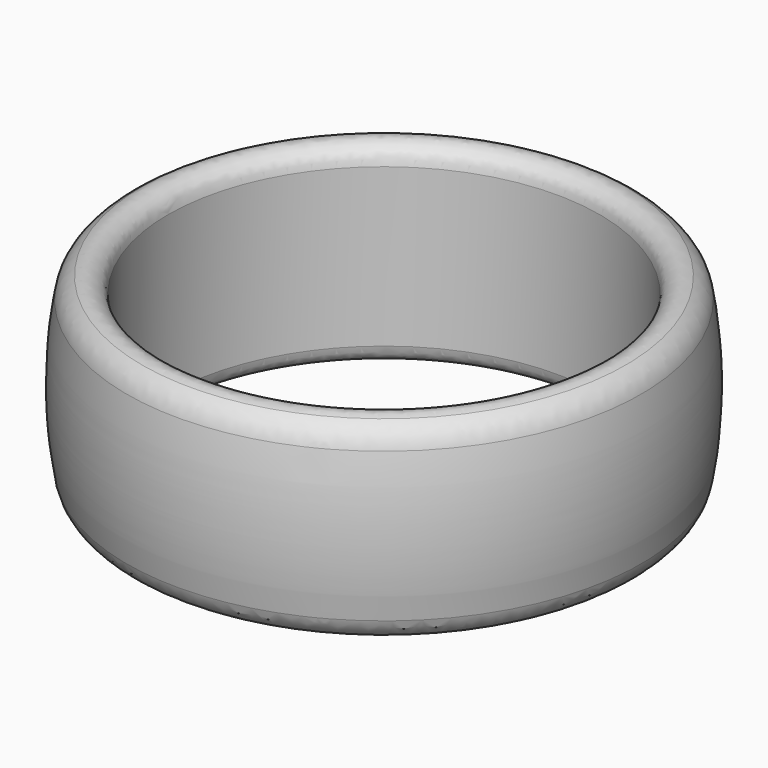
from build123d import *

# Parameters (mm, degrees)
F0_R          = 9
F1_DEPTH      = 5
F4_R          = 1.2
F5_R          = 0.75
F8_W          = 4.5
F8_H          = 1
F8_W_2        = 1
F8_H_2        = 4.5
F9_DEPTH      = 6.4
F10_TEXT_SIZE = 5.5555555556
F11_DEPTH     = 1
F12_TEXT_SIZE = 5.5555555556
F13_DEPTH     = 1
F14_TEXT_SIZE = 5.5555555556
F15_DEPTH     = 1


# Not quite as in the source:
# - Text() gives the source's letters only with a copy of the font that has no kerning and outlines rounded to 1/6400 em; it was checked with that copy


with BuildPart() as f1:
    # F0 (on Top) → F1 (new body)
    with BuildSketch(Plane.XY):
        Circle(F0_R)
    extrude(amount=F1_DEPTH)


with BuildPart() as f3:
    # F2 (on Front) → F3 (revolve)
    with BuildSketch(Plane.XZ):
        with BuildLine():
            Line((-10.5, 0), (-9, 0))
            Line((-9, 0), (-9, 8.1769345951))
            Line((-9, 8.1769345951), (-10.5, 8.1769345951))
            add(Edge.make_bspline(
                [(-10.5, 8.1769345951), (-11.6867599635, 4.0884672976), (-10.5, 0)],
                knots=[0.8438243034, 0.8438243034, 0.8438243034, 2.2977683502, 2.2977683502, 2.2977683502], degree=2, weights=[1, 0.7471902488, 1]))
        make_face()
    revolve(axis=Axis((0, 0, 0), (0, 0, -1)))

    # F4
    f4_edges = [f3.edges().sort_by_distance(p)[0] for p in [
        (10.5, 0, 8.176935),
        (10.5, 0, 0),
    ]]
    fillet(f4_edges, radius=F4_R)

    # F5
    f5_edges = [f3.edges().sort_by_distance(p)[0] for p in [
        (9, 0, 0),
        (9, 0, 8.176935),
    ]]
    fillet(f5_edges, radius=F5_R)

    # F8 (on offset) → F9 (join)
    with BuildSketch(Plane.XY.offset(7)):
        with Locations((0, -9.8633077815)):
            Rectangle(F8_W, F8_H)
        Polygon((6.6302110493, -6.9838624022), (2.7330967322, -9.2338624022), (3.2330967322, -10.099887806), (7.1302110493, -7.849887806), align=None)
        Polygon((9.2338624022, -2.7330967322), (6.9838624022, -6.6302110493), (7.849887806, -7.1302110493), (10.099887806, -3.2330967322), align=None)
        with Locations((9.8633077815, 0)):
            Rectangle(F8_W_2, F8_H_2)
        Polygon((6.9838624022, 6.6302110493), (9.2338624022, 2.7330967322), (10.099887806, 3.2330967322), (7.849887806, 7.1302110493), align=None)
        Polygon((2.7330967322, 9.2338624022), (6.6302110493, 6.9838624022), (7.1302110493, 7.849887806), (3.2330967322, 10.099887806), align=None)
        with Locations((0, 9.8633077815)):
            Rectangle(F8_W, F8_H)
        Polygon((-6.6302110493, 6.9838624022), (-2.7330967322, 9.2338624022), (-3.2330967322, 10.099887806), (-7.1302110493, 7.849887806), align=None)
        Polygon((-9.2338624022, 2.7330967322), (-6.9838624022, 6.6302110493), (-7.849887806, 7.1302110493), (-10.099887806, 3.2330967322), align=None)
        with Locations((-9.8633077815, 0)):
            Rectangle(F8_W_2, F8_H_2)
        Polygon((-6.9838624022, -6.6302110493), (-9.2338624022, -2.7330967322), (-10.099887806, -3.2330967322), (-7.849887806, -7.1302110493), align=None)
        Polygon((-2.7330967322, -9.2338624022), (-6.6302110493, -6.9838624022), (-7.1302110493, -7.849887806), (-3.2330967322, -10.099887806), align=None)
    extrude(amount=-F9_DEPTH)

    # F10 (on face) → F11 (cut)
    with BuildSketch(Plane(origin=(0, 10.3633077815, 0), x_dir=(-1, 0, 0), z_dir=(0, 1, 0))):
        with Locations((-1.3956547633, 1.974224723)):
            Text('F', F10_TEXT_SIZE, font='Open Sans', font_style=FontStyle.BOLD, text_align=(TextAlign.LEFT, TextAlign.BOTTOM))
    extrude(amount=F11_DEPTH, mode=Mode.SUBTRACT)

    # F12 (on face) → F13 (cut)
    with BuildSketch(Plane(origin=(-5.1816538908, 8.974887806, 0), x_dir=(-0.8660254038, -0.5, 0), z_dir=(-0.5, 0.8660254038, 0))):
        with Locations((-1.9036158307, 1.974224723)):
            Text('C', F12_TEXT_SIZE, font='Open Sans', font_style=FontStyle.BOLD, text_align=(TextAlign.LEFT, TextAlign.BOTTOM))
    extrude(amount=F13_DEPTH, mode=Mode.SUBTRACT)

    # F14 (on face) → F15 (cut)
    with BuildSketch(Plane(origin=(-8.974887806, 5.1816538908, 0), x_dir=(-0.5, -0.8660254038, 0), z_dir=(-0.8660254038, 0.5, 0))):
        with Locations((-1.4044659477, 1.974224723)):
            Text('A', F14_TEXT_SIZE, font='Open Sans', font_style=FontStyle.BOLD, text_align=(TextAlign.LEFT, TextAlign.BOTTOM))
    extrude(amount=F15_DEPTH, mode=Mode.SUBTRACT)


solid = f3.part
